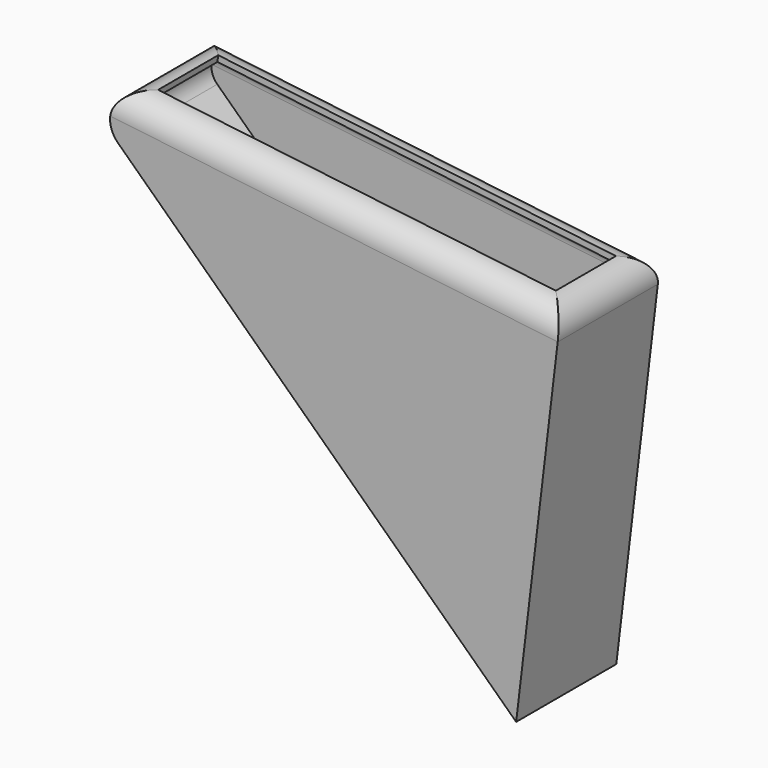
from build123d import *

# Parameters (mm, degrees)
F1_DEPTH = 25.4
F2_R     = 5.08
F3_T     = -1.27


# Not quite as in the source:
# - a shell that OpenCascade refuses in one call is made with other operations: the cavity is built on its own and cut out


with BuildPart() as f1:
    # F0 (on Front) → F1 (new body)
    with BuildSketch(Plane.XZ):
        Polygon((-9.891229794, 75.6632118021), (-110.7755121968, 87.7015490657), (-18.9199827418, 0), align=None)
    extrude(amount=-F1_DEPTH)

    # F2
    f2_edges = [f1.edges().sort_by_distance(p)[0] for p in [
        (-60.333371, 0, 81.68238),
        (-110.775512, 12.7, 87.701549),
        (-60.333371, 25.4, 81.68238),
        (-9.89123, 12.7, 75.663212),
    ]]
    fillet(f2_edges, radius=F2_R)

    # F3: a shell. OpenCascade refuses it in one call, so the cavity is built on its own and cut out:
    # the body offset inwards by the wall thickness, plus a prism from it out through each open face.
    f3_core = offset(f1.part, amount=F3_T, mode=Mode.PRIVATE)
    f3_exits = [f3_core.faces().sort_by_distance(p)[0] for p in [
        (-55.439636, 12.7, 79.81941),
    ]]
    add(f3_core, mode=Mode.SUBTRACT)
    extrude(f3_exits, amount=-F3_T, mode=Mode.SUBTRACT)


solid = f1.part
